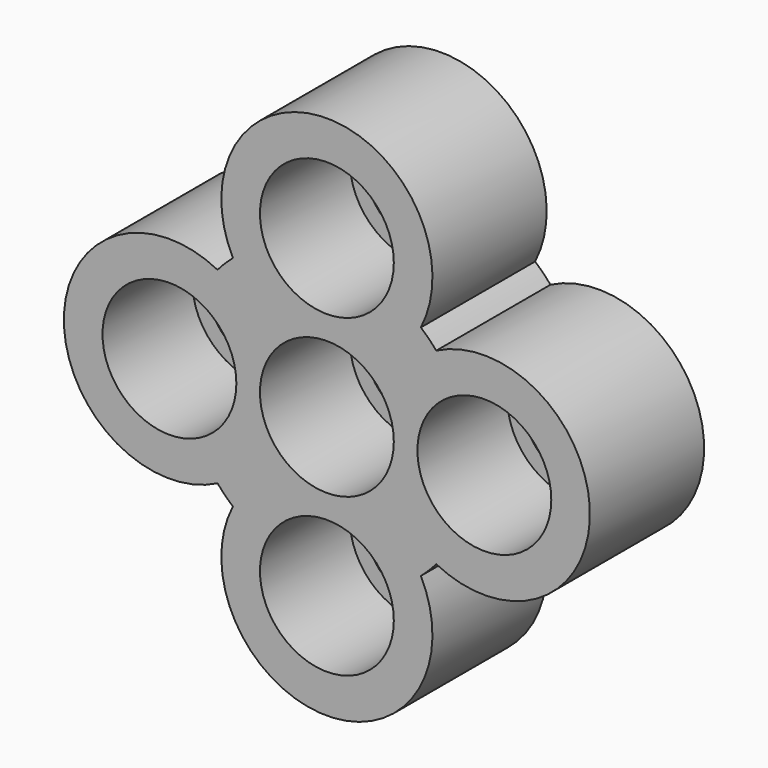
from build123d import *

# Parameters (mm, degrees)
F0_R     = 11
F1_DEPTH = 18.4658
F2_DEPTH = 5
F3_R     = 8.382
F4_DEPTH = 25.4


# Not quite as in the source:
# - a feature of the source that left no trace in its solid (it failed there, or was rolled back) is left out


with BuildPart() as f1:
    # F0 (on Front) → F1 (new body)
    with BuildSketch(Plane.XZ):
        with BuildLine():
            ThreePointArc((17.9760799845, 15.4450816893), (16.7584308008, 16.7584306274), (15.4450818753, 17.9760798247))
            ThreePointArc((15.4450818753, 17.9760798247), (0, 43.2300002384), (-15.4450818753, 17.9760798247))
            ThreePointArc((-15.4450818753, 17.9760798247), (-16.7584308008, 16.7584306274), (-17.9760799845, 15.4450816893))
            ThreePointArc((-17.9760799845, 15.4450816893), (-43.23, 0), (-17.9760799845, -15.4450816893))
            ThreePointArc((-17.9760799845, -15.4450816893), (-16.7584307141, -16.7584307141), (-15.4450816893, -17.9760799845))
            ThreePointArc((-15.4450816893, -17.9760799845), (0, -43.23), (15.4450816893, -17.9760799845))
            ThreePointArc((15.4450816893, -17.9760799845), (16.7584307141, -16.7584307141), (17.9760799845, -15.4450816893))
            ThreePointArc((17.9760799845, -15.4450816893), (43.23, 0), (17.9760799845, 15.4450816893))
        make_face()
        with Locations((-25.88, 0)):
            Circle(F0_R, mode=Mode.SUBTRACT)
        with Locations((0, -25.88)):
            Circle(F0_R, mode=Mode.SUBTRACT)
        Circle(F0_R, mode=Mode.SUBTRACT)
        with Locations((25.88, 0)):
            Circle(F0_R, mode=Mode.SUBTRACT)
        with Locations((0, 25.88)):
            Circle(F0_R, mode=Mode.SUBTRACT)
    extrude(amount=F1_DEPTH)

    # F0 (on Front) → F2 (join)
    with BuildSketch(Plane.XZ):
        with BuildLine():
            ThreePointArc((17.9760799845, 15.4450816893), (16.7584308008, 16.7584306274), (15.4450818753, 17.9760798247))
            ThreePointArc((15.4450818753, 17.9760798247), (0, 43.2300002384), (-15.4450818753, 17.9760798247))
            ThreePointArc((-15.4450818753, 17.9760798247), (-16.7584308008, 16.7584306274), (-17.9760799845, 15.4450816893))
            ThreePointArc((-17.9760799845, 15.4450816893), (-43.23, 0), (-17.9760799845, -15.4450816893))
            ThreePointArc((-17.9760799845, -15.4450816893), (-16.7584307141, -16.7584307141), (-15.4450816893, -17.9760799845))
            ThreePointArc((-15.4450816893, -17.9760799845), (0, -43.23), (15.4450816893, -17.9760799845))
            ThreePointArc((15.4450816893, -17.9760799845), (16.7584307141, -16.7584307141), (17.9760799845, -15.4450816893))
            ThreePointArc((17.9760799845, -15.4450816893), (43.23, 0), (17.9760799845, 15.4450816893))
        make_face()
        with Locations((-25.88, 0)):
            Circle(F0_R, mode=Mode.SUBTRACT)
        with Locations((0, -25.88)):
            Circle(F0_R, mode=Mode.SUBTRACT)
        Circle(F0_R, mode=Mode.SUBTRACT)
        with Locations((25.88, 0)):
            Circle(F0_R, mode=Mode.SUBTRACT)
        with Locations((0, 25.88)):
            Circle(F0_R, mode=Mode.SUBTRACT)
        with Locations((0, 25.88)):
            Circle(F0_R)
        with Locations((25.88, 0)):
            Circle(F0_R)
        Circle(F0_R)
        with Locations((-25.88, 0)):
            Circle(F0_R)
        with Locations((0, -25.88)):
            Circle(F0_R)
    extrude(amount=-F2_DEPTH)

    # F3 (on face) → F4 (cut)
    with BuildSketch(Plane(origin=(0, 5, 0), x_dir=(-1, 0, 0), z_dir=(0, 1, 0))):
        with Locations((0, 25.88)):
            Circle(F3_R)
        with Locations((-25.88, 0)):
            Circle(F3_R)
        Circle(F3_R)
        with Locations((0, -25.88)):
            Circle(F3_R)
        with Locations((25.88, 0)):
            Circle(F3_R)
    extrude(amount=-F4_DEPTH, mode=Mode.SUBTRACT)


solid = f1.part
